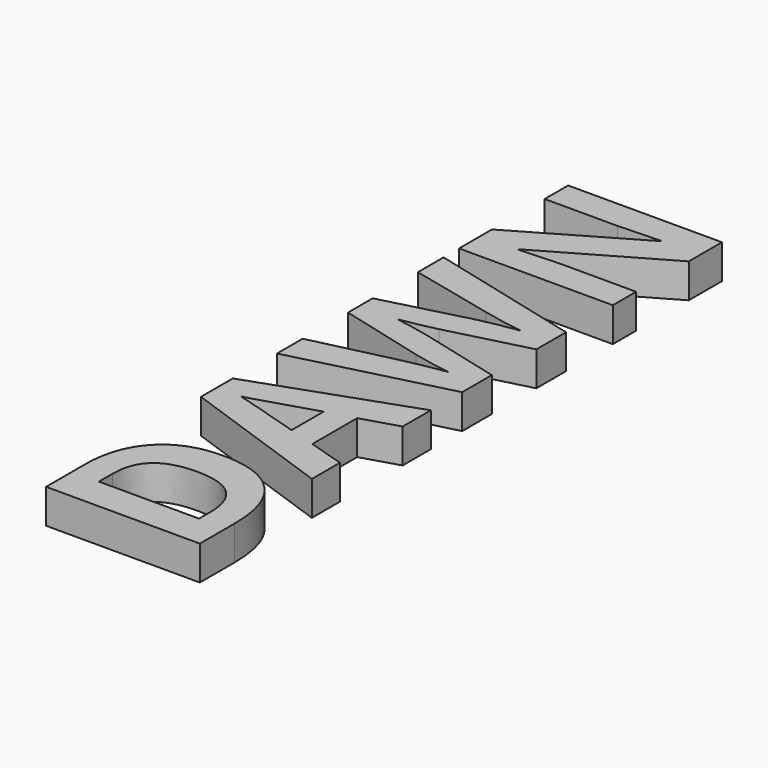
from build123d import *

# Parameters (mm, degrees)
F0_TEXT_SIZE = 12.5582536179
F1_DEPTH     = 2


# Not quite as in the source:
# - Text() gives the source's letters only with a copy of the font that has no kerning and outlines rounded to 1/6400 em; it was checked with that copy


with BuildPart() as f1:
    # F0 (on Top) → F1 (new body)
    with BuildSketch(Plane.XY):
        with Locations(Location((0, 0.0127404056), (0, 0, 90))):
            Text('DAWN', F0_TEXT_SIZE, font='Open Sans', font_style=FontStyle.BOLD, text_align=(TextAlign.LEFT, TextAlign.BOTTOM))
    extrude(amount=F1_DEPTH)


solid = f1.part
